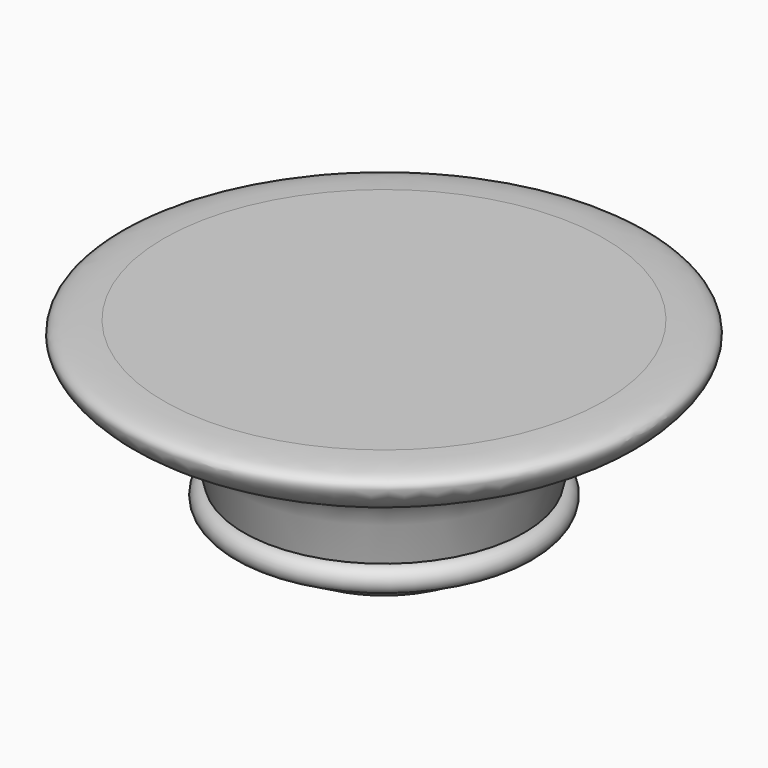
from build123d import *


with BuildPart() as f1:
    # F0 (on Front) → F1 (revolve)
    with BuildSketch(Plane.XZ):
        with BuildLine():
            Line((0, 70.1842084527), (0, 0))
            Line((0, 0), (22.7396823466, 0))
            add(Edge.make_bspline(
                [(22.7396823466, 0), (31.3707231713, 3.9517153813), (40.001763996, 7.9034307625), (44.5460036318, 14.9970185966)],
                knots=[0, 0, 0, 0, 0.2115090405, 0.2115090405, 0.2115090405, 0.2115090405], degree=3))
            add(Edge.make_bspline(
                [(44.5460036318, 14.9970185966), (44.8174749118, 15.4207870426), (46.0982067573, 17.5894295368), (46.994751399, 20.0534294847), (47.5912563159, 22.1146519768)],
                knots=[0.2115090405, 0.2115090405, 0.2115090405, 0.2115090405, 0.2241445163, 0.2745044692, 0.2745044692, 0.2745044692, 0.2745044692], degree=3))
            add(Edge.make_bspline(
                [(47.5912563159, 22.1146519768), (49.663673869, 29.2758899683), (51.1134227247, 48.5590309681), (81.5962278167, 52.7939949916), (94.1960510541, 69.6562341921), (81.3245532577, 70.0043798994), (74.6760070324, 70.1842084527)],
                knots=[0.2745044692, 0.2745044692, 0.2745044692, 0.2745044692, 0.449468409, 0.6827123966, 0.8361106585, 1, 1, 1, 1], degree=3))
            Line((74.6760070324, 70.1842084527), (0, 70.1842084527))
        make_face()
        with BuildLine():
            add(Edge.make_bspline(
                [(44.5460036318, 14.9970185966), (44.8174749118, 15.4207870426), (46.0982067573, 17.5894295368), (46.994751399, 20.0534294847), (47.5912563159, 22.1146519768)],
                knots=[0.2115090405, 0.2115090405, 0.2115090405, 0.2115090405, 0.2241445163, 0.2745044692, 0.2745044692, 0.2745044692, 0.2745044692], degree=3))
            ThreePointArc((44.5460036318, 14.9970185966), (51.2693875538, 16.3307107075), (47.5912563159, 22.1146519768))
        make_face()
    revolve(axis=Axis((0, 0, 35.0921042264), (0, 0, 1)))


solid = f1.part
